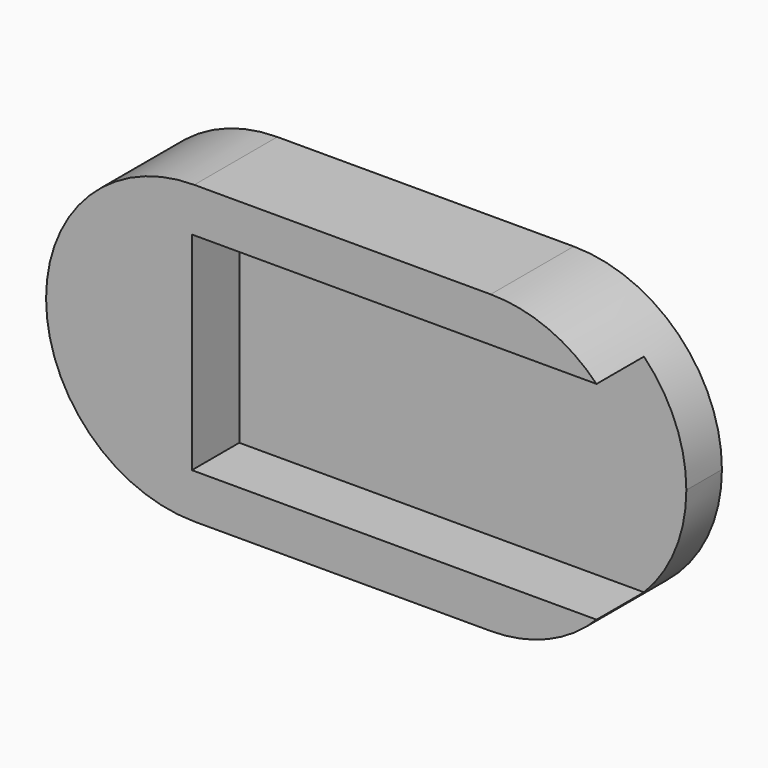
from build123d import *

# Parameters (mm, degrees)
F1_DEPTH     = 7
F3_DEPTH     = 4
F4_TEXT_SIZE = 13.8888888889
F5_DEPTH     = 0.5


# Not quite as in the source:
# - Text() gives the source's letters only with a copy of the font that has no kerning and outlines rounded to 1/6400 em; it was checked with that copy


with BuildPart() as f1:
    # F0 (on Front) → F1 (new body)
    with BuildSketch(Plane.XZ):
        with BuildLine():
            ThreePointArc((-29.8368941145, -10), (-22.7658263026, -7.0710678119), (-19.8368941145, 0))
            ThreePointArc((-19.8368941145, 0), (-22.7658263026, 7.0710678119), (-29.8368941145, 10))
            ThreePointArc((-29.8368941145, 10), (-39.8368941145, 0), (-29.8368941145, -10))
        make_face()
        with BuildLine():
            ThreePointArc((-29.8368941145, 10), (-22.7658263026, 7.0710678119), (-19.8368941145, 0))
            ThreePointArc((-19.8368941145, 0), (-16.9079619263, 7.0710678119), (-9.8368941145, 10))
            Line((-9.8368941145, 10), (-29.8368941145, 10))
        make_face()
        with BuildLine():
            ThreePointArc((-9.8368941145, 10), (-16.9079619263, 7.0710678119), (-19.8368941145, 0))
            ThreePointArc((-19.8368941145, 0), (-16.9079619263, -7.0710678119), (-9.8368941145, -10))
            ThreePointArc((-9.8368941145, -10), (-2.7658263026, -7.0710678119), (0.1631058855, 0))
            ThreePointArc((0.1631058855, 0), (-2.7658263026, 7.0710678119), (-9.8368941145, 10))
        make_face()
        with BuildLine():
            ThreePointArc((-9.8368941145, -10), (-16.9079619263, -7.0710678119), (-19.8368941145, 0))
            ThreePointArc((-19.8368941145, 0), (-22.7658263026, -7.0710678119), (-29.8368941145, -10))
            Line((-29.8368941145, -10), (-9.8368941145, -10))
        make_face()
    extrude(amount=F1_DEPTH)

    # F2 (on face) → F3 (cut)
    with BuildSketch(Plane.XZ.offset(7)):
        with BuildLine():
            Line((30, 7), (-2.6954656859, 7))
            ThreePointArc((-2.6954656859, 7), (0.1631058855, 0), (-2.6954656859, -7))
            Line((-2.6954656859, -7), (30, -7))
            Line((30, -7), (30, 7))
        make_face()
        with BuildLine():
            Line((-2.6954656859, 7), (-30, 7))
            Line((-30, 7), (-30, -7))
            Line((-30, -7), (-2.6954656859, -7))
            ThreePointArc((-2.6954656859, -7), (0.1631058855, 0), (-2.6954656859, 7))
        make_face()
    extrude(amount=-F3_DEPTH, mode=Mode.SUBTRACT)

    # F4 (on face) → F5 (join)
    with BuildSketch(Plane(origin=(0, 0, 0), x_dir=(-1, 0, 0), z_dir=(0, 1, 0))):
        with Locations((9.8368941145, -5)):
            Text('MD', F4_TEXT_SIZE, font='Open Sans', text_align=(TextAlign.LEFT, TextAlign.BOTTOM))
    extrude(amount=F5_DEPTH)


solid = f1.part
